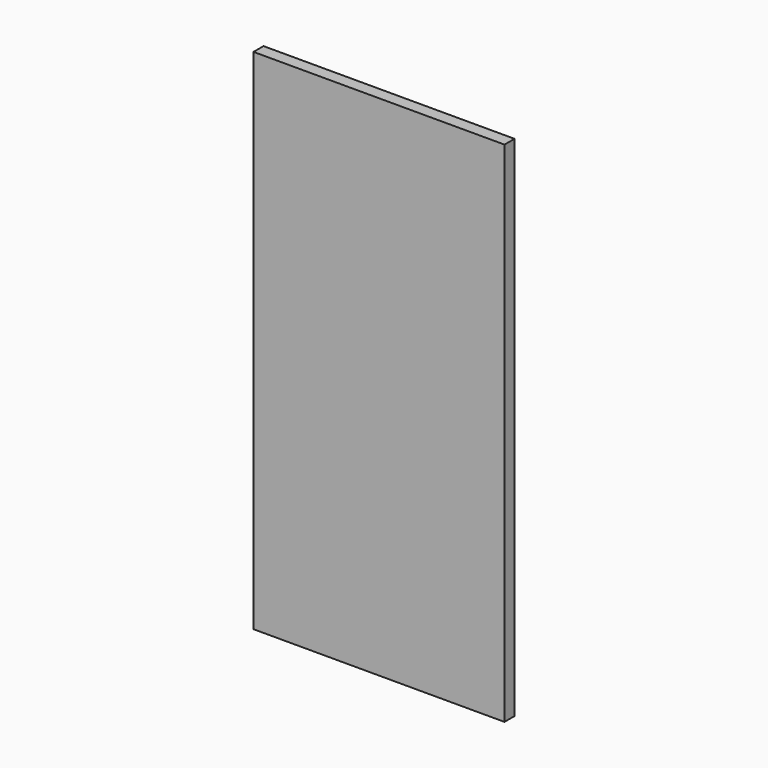
from build123d import *

# Parameters (mm, degrees)
F0_W     = 63.5
F0_H     = 128.5776956
F1_DEPTH = 3.175


# Not quite as in the source:
# - a length typed as a fraction of an inch, garbled in the dataset ("3 / 203.2 mm" for 3/8 in), is restored


with BuildPart() as f1:
    # F0 (on Front) → F1 (new body)
    with BuildSketch(Plane.XZ):
        Rectangle(F0_W, F0_H)
    extrude(amount=F1_DEPTH)


solid = f1.part
